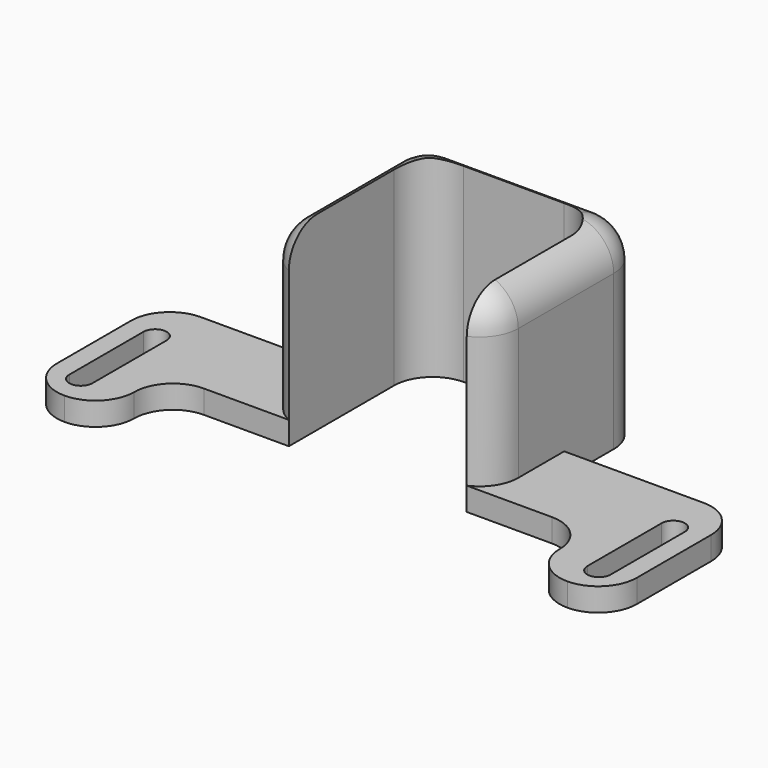
from build123d import *

# Parameters (mm, degrees)
F2_DEPTH     = 25
F3_DEPTH     = 3
F4_DEPTH     = 25
F5_R         = 4.99999
F6_T1_DEPTH  = 25
F6_T3_DEPTH  = 25
F6_T5_DEPTH  = 50
F6_T7_DEPTH  = 33.4564392374
F6_T9_DEPTH  = 50
F6_T11_DEPTH = 33.4564392374
F7_T1_DEPTH  = 15.417424305
F7_T3_DEPTH  = 19
F7_T6_ANGLE  = 89.9999999974
F7_T8_ANGLE  = 89.9999999974
F7_T10_ANGLE = 209.6926070845
F7_T12_ANGLE = 209.6926070845


# Not quite as in the source:
# - a fillet or chamfer that OpenCascade refuses, or shapes differently, is made with other operations: its cross-section is extruded or revolved along the edge and cut away or added
# - a fillet or chamfer is up to 0.001 mm smaller than in the source, because OpenCascade refuses the exact size


with BuildPart() as f2:
    # F0 (on Top) → F2 (new body)
    with BuildSketch(Plane.XY):
        Polygon((14.5, 35), (0, 35), (-14.5, 35), (-14.5, 22), (-14.5, 10), (-11.5, 10), (-11.5, 32), (0, 32), (11.5, 32), (11.5, 10), (14.5, 10), (14.5, 22), align=None)
    extrude(amount=F2_DEPTH)

    # F0 (on Top) → F3 (join)
    with BuildSketch(Plane.XY):
        Polygon((-14.5, 10), (-14.5, 22), (-37.5, 22), (-37.5, 0), (-27.5, 0), (-27.5, 10), align=None)
        Polygon((37.5, 22), (14.5, 22), (14.5, 10), (27.5, 10), (27.5, 0), (37.5, 0), align=None)
    extrude(amount=F3_DEPTH)

    # F1 (on Top) → F4 (cut)
    with BuildSketch(Plane.XY):
        with BuildLine():
            Line((35, 3.8767794613), (35, 15.8767794613))
            ThreePointArc((35, 15.8767794613), (33.5, 17.3767794613), (32, 15.8767794613))
            Line((32, 15.8767794613), (32, 3.8767794613))
            ThreePointArc((32, 3.8767794613), (33.5, 2.3767794613), (35, 3.8767794613))
        make_face()
        with BuildLine():
            ThreePointArc((-32, 15.8767794613), (-33.5, 17.3767794613), (-35, 15.8767794613))
            Line((-35, 15.8767794613), (-35, 3.8767794613))
            ThreePointArc((-35, 3.8767794613), (-33.5, 2.3767794613), (-32, 3.8767794613))
            Line((-32, 3.8767794613), (-32, 15.8767794613))
        make_face()
    extrude(amount=F4_DEPTH, mode=Mode.SUBTRACT)

    # F5 (radius 5 in the source; OpenCascade refuses exactly that, so slightly less here)
    f5_edges = [f2.edges().sort_by_distance(p)[0] for p in [
        (-37.5, 0, 1.5),
        (-27.5, 0, 1.5),
        (-37.5, 22, 1.5),
        (37.5, 22, 1.5),
        (37.5, 0, 1.5),
        (27.5, 0, 1.5),
        (27.5, 10, 1.5),
        (-27.5, 10, 1.5),
    ]]
    fillet(f5_edges, radius=F5_R)

    # F6: fillet of radius 5 on 6 edges, made by hand

    # F6_s2 → F6_t1 (join)
    with BuildSketch(Plane.XY):
        with BuildLine():
            ThreePointArc((11.5, 27), (10.0355339059, 30.5355339059), (6.5, 32))
            Line((6.5, 32), (11.5, 32))
            Line((11.5, 32), (11.5, 27))
        make_face()
    extrude(amount=F6_T1_DEPTH)

    # F6_s4 → F6_t3 (join)
    with BuildSketch(Plane.XY):
        with BuildLine():
            ThreePointArc((-6.5, 32), (-10.0355339059, 30.5355339059), (-11.5, 27))
            Line((-11.5, 27), (-11.5, 32))
            Line((-11.5, 32), (-6.5, 32))
        make_face()
    extrude(amount=F6_T3_DEPTH)

    # F6_s6 → F6_t5 (cut)
    with BuildSketch(Plane.XY.offset(-12.5)):
        with BuildLine():
            ThreePointArc((14.5, 30), (13.0355339059, 33.5355339059), (9.5, 35))
            Line((9.5, 35), (14.5, 35))
            Line((14.5, 35), (14.5, 30))
        make_face()
    extrude(amount=F6_T5_DEPTH, mode=Mode.SUBTRACT)

    # F6_s8 → F6_t7 (cut)
    with BuildSketch(Plane.XY.offset(3)):
        with BuildLine():
            ThreePointArc((11.5, 10), (13.6833001327, 11.8439629074), (14.5, 14.582575695))
            Line((14.5, 14.582575695), (14.5, 10))
            Line((14.5, 10), (11.5, 10))
        make_face()
    extrude(amount=F6_T7_DEPTH, mode=Mode.SUBTRACT)

    # F6_s10 → F6_t9 (cut)
    with BuildSketch(Plane.XY.offset(-12.5)):
        with BuildLine():
            ThreePointArc((-9.5, 35), (-13.0355339059, 33.5355339059), (-14.5, 30))
            Line((-14.5, 30), (-14.5, 35))
            Line((-14.5, 35), (-9.5, 35))
        make_face()
    extrude(amount=F6_T9_DEPTH, mode=Mode.SUBTRACT)

    # F6_s12 → F6_t11 (cut)
    with BuildSketch(Plane.XY.offset(3)):
        with BuildLine():
            ThreePointArc((-11.5, 10), (-13.6833001327, 11.8439629074), (-14.5, 14.582575695))
            Line((-14.5, 14.582575695), (-14.5, 10))
            Line((-14.5, 10), (-11.5, 10))
        make_face()
    extrude(amount=F6_T11_DEPTH, mode=Mode.SUBTRACT)

    # F7: fillet of radius 5 on 3 edges, made by hand

    # F7_s2 → F7_t1 (cut)
    with BuildSketch(Plane.XZ.offset(-30)):
        with BuildLine():
            ThreePointArc((-9.5, 25), (-13.0355339059, 23.5355339059), (-14.5, 20))
            Line((-14.5, 20), (-14.5, 25))
            Line((-14.5, 25), (-9.5, 25))
        make_face()
        with BuildLine():
            ThreePointArc((9.5, 25), (13.0355339059, 23.5355339059), (14.5, 20))
            Line((14.5, 20), (14.5, 25))
            Line((14.5, 25), (9.5, 25))
        make_face()
    extrude(amount=F7_T1_DEPTH, mode=Mode.SUBTRACT)

    # F7_s4 → F7_t3 (cut)
    with BuildSketch(Plane.YZ.offset(-9.5)):
        with BuildLine():
            ThreePointArc((30, 25), (33.5355339059, 23.5355339059), (35, 20))
            Line((35, 20), (35, 25))
            Line((35, 25), (30, 25))
        make_face()
    extrude(amount=F7_T3_DEPTH, mode=Mode.SUBTRACT)

    # F7_s5 → F7_t6 (revolve, cut)
    with BuildSketch(Plane.YZ.offset(9.4999999999)):
        with BuildLine():
            ThreePointArc((30, 25), (33.5355339059, 23.5355339059), (35, 20))
            Line((35, 20), (35, 25))
            Line((35, 25), (30, 25))
        make_face()
    revolve(axis=Axis((9.4999999999, 29.9999999999, 25), (0, 0, -1)), revolution_arc=F7_T6_ANGLE, mode=Mode.SUBTRACT)

    # F7_s7 → F7_t8 (revolve, cut)
    with BuildSketch(Plane.XZ.offset(-29.9999999999)):
        with BuildLine():
            ThreePointArc((-9.5, 25), (-13.0355339059, 23.5355339059), (-14.5, 20))
            Line((-14.5, 20), (-14.5, 25))
            Line((-14.5, 25), (-9.5, 25))
        make_face()
    revolve(axis=Axis((-9.4999999999, 29.9999999999, 25), (0, 0, -1)), revolution_arc=F7_T8_ANGLE, mode=Mode.SUBTRACT)

    # F7_s9 → F7_t10 (revolve, cut)
    with BuildSketch(Plane.XZ.offset(-14.5825756948)):
        with BuildLine():
            ThreePointArc((14.5, 20), (13.0355339059, 23.5355339059), (9.5, 25))
            Line((9.5, 25), (14.5, 25))
            Line((14.5, 25), (14.5, 20))
        make_face()
    revolve(axis=Axis((9.5000000002, 14.5825756948, 25), (0, 0, -1)), revolution_arc=F7_T10_ANGLE, mode=Mode.SUBTRACT)

    # F7_s11 → F7_t12 (revolve, cut)
    with BuildSketch(Plane(origin=(-8.6059581245, 15.0923752984, 0), x_dir=(0, 0, 1), z_dir=(-0.4953465841, 0.8686954366, 0))):
        with BuildLine():
            ThreePointArc((25, -1.02917759), (23.5355339059, 2.506356316), (20, 3.97082241))
            Line((20, 3.97082241), (25, 3.97082241))
            Line((25, 3.97082241), (25, -1.02917759))
        make_face()
    revolve(axis=Axis((-9.5000000002, 14.5825756948, 25), (0, 0, -1)), revolution_arc=F7_T12_ANGLE, mode=Mode.SUBTRACT)


solid = f2.part
